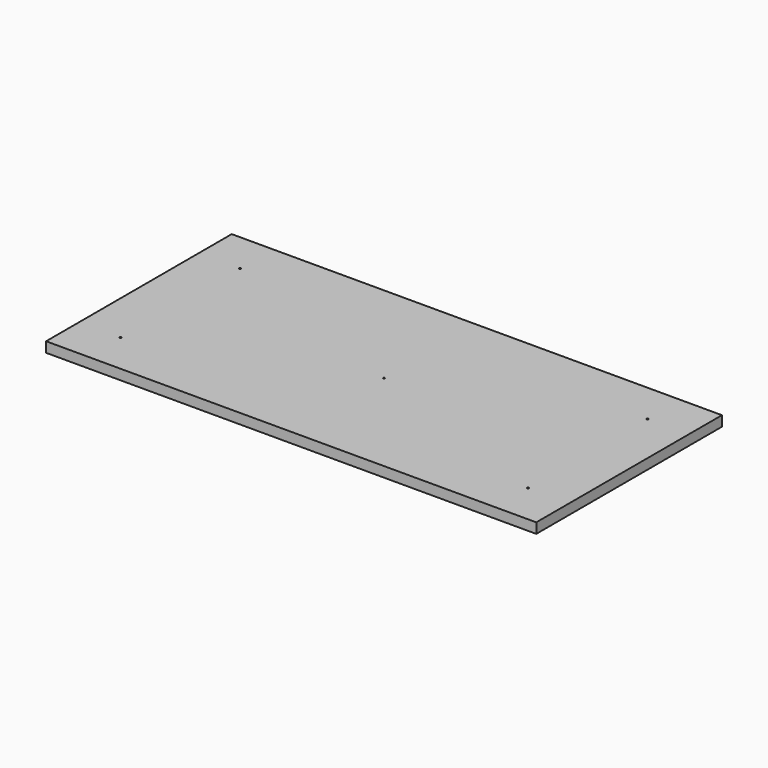
from build123d import *

# Parameters (mm, degrees)
F0_W     = 916.432
F0_H     = 433.832
F1_DEPTH = 19.05
F3_D     = 8.001
F3_DEPTH = 14.224
F3_TIP   = 2.4037429064
F5_D     = 3.175
F5_DEPTH = 20.32
F5_TIP   = 0.9538662327


with BuildPart() as f1:
    # F0 (on Top) → F1 (new body)
    with BuildSketch(Plane.XY):
        Rectangle(F0_W, F0_H)
    extrude(amount=F1_DEPTH)

    # F3
    with Locations(Plane(origin=(0, 0, 0), x_dir=(1, 0, 0), z_dir=(0, 0, -1))):
        with Locations((-448.5894, 165.1), (-448.5894, 0), (-448.5894, -165.1), (-387.35, -207.2894), (0, -207.2894), (387.35, -207.2894), (448.5894, -165.1), (448.5894, 0), (448.5894, 165.1)):
            Hole(F3_D / 2, depth=F3_DEPTH)
            with Locations((0, 0, -(F3_DEPTH + F3_TIP / 2))):  # 118° drill point
                Cone(0, F3_D / 2, F3_TIP, mode=Mode.SUBTRACT)

    # F5
    with Locations(Plane(origin=(0, 0, 0), x_dir=(1, 0, 0), z_dir=(0, 0, -1))):
        with Locations((-381, 139.7), (0, 0), (-381, -139.7), (381, -139.7), (381, 139.7)):
            Hole(F5_D / 2, depth=F5_DEPTH)
            with Locations((0, 0, -(F5_DEPTH + F5_TIP / 2))):  # 118° drill point
                Cone(0, F5_D / 2, F5_TIP, mode=Mode.SUBTRACT)


solid = f1.part
